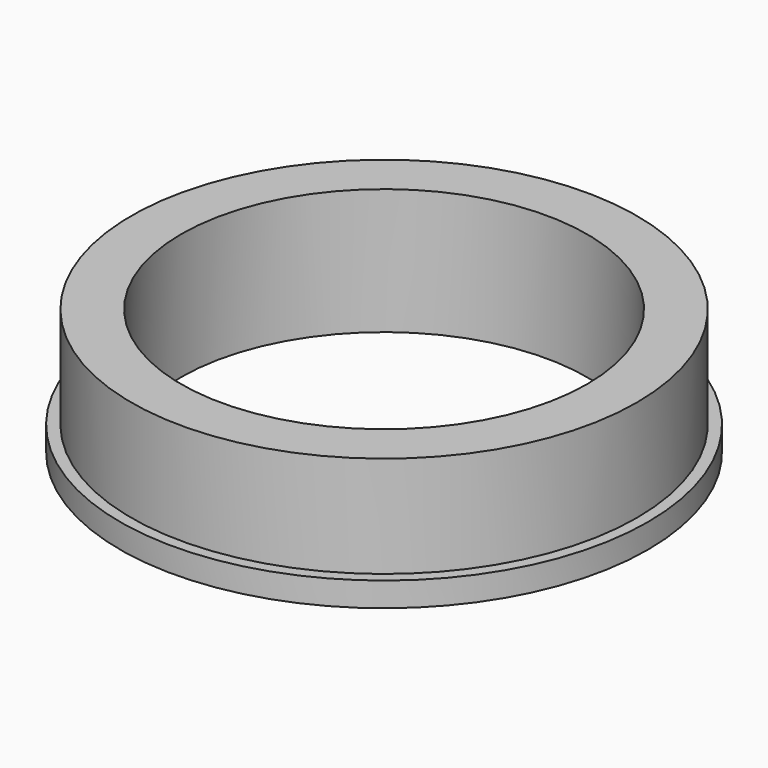
from build123d import *

# Parameters (mm, degrees)
F0_R     = 15.8115
F0_R_2   = 12.7
F1_DEPTH = 6.35
F2_R     = 16.51
F2_R_2   = 15.8115
F2_R_3   = 12.7
F3_DEPTH = 1.524


with BuildPart() as f1:
    # F0 (on Top) → F1 (new body)
    with BuildSketch(Plane.XY):
        Circle(F0_R)
        Circle(F0_R_2, mode=Mode.SUBTRACT)
    extrude(amount=F1_DEPTH)

    # F2 (on face) → F3 (join)
    with BuildSketch(Plane(origin=(0, 0, 0), x_dir=(1, 0, 0), z_dir=(0, 0, -1))):
        Circle(F2_R)
        Circle(F2_R_2, mode=Mode.SUBTRACT)
        Circle(F2_R_2)
        Circle(F2_R_3, mode=Mode.SUBTRACT)
    extrude(amount=F3_DEPTH)


solid = f1.part
